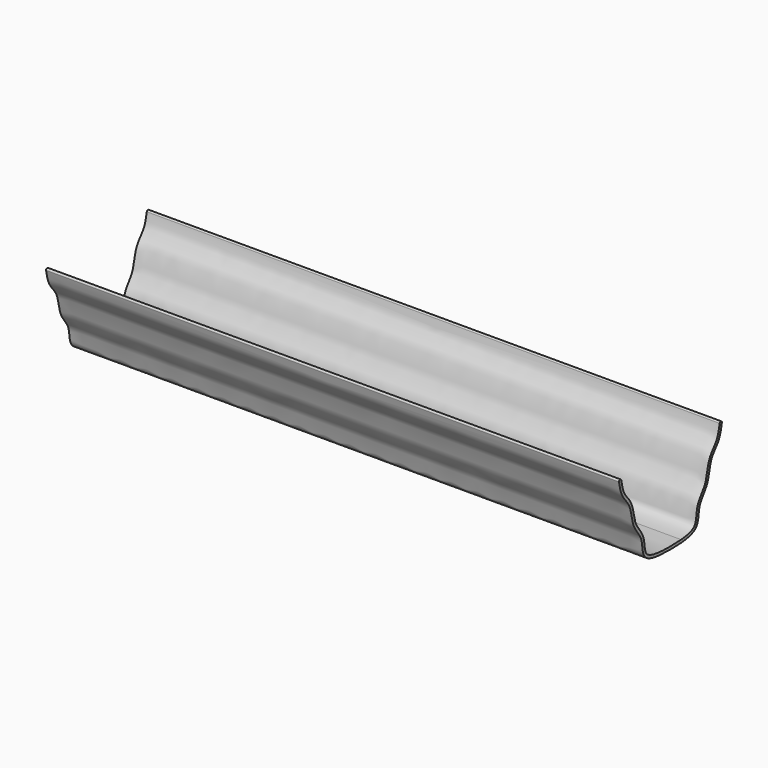
from build123d import *

# Parameters (mm, degrees)
F1_DEPTH = 610


# Not quite as in the source:
# - ends of sketch curves that miss each other by under 0.0002 mm in the source are joined
# - the dataset's text gives a spline's control points without its knots; the knots are read off the source's solid


with BuildPart() as f1:
    # F0 (on Right) → F1 (new body)
    with BuildSketch(Plane.YZ):
        with BuildLine():
            add(Edge.make_bspline(
                [(-6.5371447453, 100.0838043479), (-6.7706498844, 98.7103560222), (-7.2769413201, 95.966442744), (-8.2462300011, 91.9595019059), (-9.3037510376, 88.7948658007), (-10.3440569893, 86.4178038959), (-11.2307456768, 84.7238978183), (-12.2403989924, 83.1327544504), (-13.7314030487, 81.0971306843), (-15.7697396376, 78.6342860816), (-17.8019003352, 76.0598448924), (-19.2697771779, 73.7976975728), (-20.2543484515, 71.9667309835), (-21.0728069506, 69.9675927938), (-21.9644751836, 67.1317082104), (-22.8208505479, 63.3393291587), (-23.5880679523, 59.4204357255), (-24.2982442677, 56.3341514977), (-24.9152930999, 54.0757040586), (-25.5299125954, 52.2670731086), (-26.0987925353, 50.8798986568), (-26.7265419191, 49.5377250168), (-27.6192869804, 47.9259926379), (-28.8144352862, 46.0694225719), (-30.0870954542, 44.2604615596), (-31.3889305982, 42.4695513152), (-32.6711410298, 40.6663234118), (-33.8840399285, 38.8197513275), (-34.9770680963, 36.8983087952), (-35.7441787823, 35.2087841297), (-36.245684668, 33.7892000703), (-36.6603912488, 32.3205401383), (-37.0314295875, 30.4232254421), (-37.3426701, 28.0880308878), (-37.7016109413, 24.956073947), (-38.2751198805, 21.1168701085), (-39.5879465674, 17.6919434206), (-41.4132093167, 15.3464026837), (-43.884361824, 13.3003757024), (-48.4648476434, 11.3486413482), (-54.6911472323, 10.0868951516), (-58.9601875507, 9.6146321059), (-60.5720902436, 9.4757778746)],
                knots=[0, 0, 0, 0, 0.03125, 0.0625, 0.09375, 0.109375, 0.125, 0.140625, 0.15625, 0.1875, 0.21875, 0.234375, 0.25, 0.265625, 0.28125, 0.3125, 0.34375, 0.359375, 0.375, 0.390625, 0.3984375, 0.40625, 0.421875, 0.4375, 0.453125, 0.46875, 0.484375, 0.5, 0.515625, 0.53125, 0.5390625, 0.546875, 0.5625, 0.578125, 0.59375, 0.625, 0.65625, 0.671875, 0.6875, 0.71875, 0.75, 0.7681993638, 0.7681993638, 0.7681993638, 0.7681993638], degree=3))
            ThreePointArc((-6.5371447453, 100.0838043479), (-7.7645113289, 101.8139967008), (-9.4947036818, 100.5866301172))
            add(Edge.make_bspline(
                [(-9.4947036818, 100.5866301172), (-9.723489658, 99.2409393238), (-10.2154650316, 96.5775155495), (-10.984099453, 93.4060678093), (-11.7253161057, 91.0179222177), (-12.351032201, 89.3152360524), (-12.9364195699, 87.9786891729), (-13.445069822, 86.9641431497), (-13.8449752198, 86.237110404), (-14.2714951974, 85.5325548459), (-14.883703547, 84.6020829341), (-15.7352720489, 83.4380223818), (-16.8740485904, 82.0050765428), (-18.0941724522, 80.5130147466), (-19.3606115163, 78.9279555444), (-20.4182743502, 77.4990743402), (-21.2400483814, 76.2738452745), (-21.8370919113, 75.3102683333), (-22.4086512808, 74.2972930377), (-22.9492281356, 73.2237773821), (-23.4401123128, 72.1063379574), (-24.0242674729, 70.5860968403), (-24.6327831857, 68.64688946), (-25.2296829702, 66.2937826991), (-25.7451190854, 63.9292340336), (-26.2217625213, 61.5819904015), (-26.6985692792, 59.280556009), (-27.2107834687, 57.056451861), (-27.6926120569, 55.295580755), (-28.1236953584, 53.960179636), (-28.473009584, 52.9974452444), (-28.8479928364, 52.0836294372), (-29.3934828733, 50.9171718759), (-30.1894656071, 49.4774115594), (-31.2965609822, 47.7557860025), (-32.5198063414, 46.0161067231), (-33.8170759051, 44.2313930138), (-35.140653965, 42.37078801), (-36.43738975, 40.3984692762), (-37.4456660647, 38.6286705807), (-38.1730927218, 37.1189779146), (-38.5863632984, 36.1338877597), (-38.8873866246, 35.3191685524), (-39.0976860325, 34.6916248477), (-39.2882860981, 34.0554206664), (-39.5152977744, 33.2063939821), (-39.7518092025, 32.1482507218), (-40.0512888446, 30.478702112), (-40.3223470736, 28.4366280651), (-40.5908821572, 26.094352671), (-40.89399031, 23.9016800338), (-41.3011875448, 21.9112530753), (-41.8613191997, 20.1758141026), (-42.6066042503, 18.7044565974), (-43.4154210799, 17.6672121122), (-44.2460282782, 16.9035328467), (-44.9853969828, 16.3577743125), (-45.8907269157, 15.8235872099), (-46.9721354151, 15.3045309126), (-48.2104811138, 14.8152141046), (-50.0529843689, 14.2110000128), (-52.6812922381, 13.5577191822), (-56.2490599407, 12.9455882658), (-59.0331081681, 12.6252377637), (-60.5727693793, 12.4869516331), (-60.7761499105, 12.4693210267)],
                knots=[0, 0, 0, 0, 0.03125, 0.0625, 0.078125, 0.09375, 0.109375, 0.1171875, 0.125, 0.1328125, 0.140625, 0.15625, 0.171875, 0.1875, 0.203125, 0.21875, 0.2265625, 0.234375, 0.2421875, 0.25, 0.2578125, 0.265625, 0.28125, 0.296875, 0.3125, 0.328125, 0.34375, 0.359375, 0.375, 0.3828125, 0.390625, 0.3984375, 0.40625, 0.421875, 0.4375, 0.453125, 0.46875, 0.484375, 0.5, 0.515625, 0.5234375, 0.53125, 0.53515625, 0.5390625, 0.54296875, 0.546875, 0.5546875, 0.5625, 0.578125, 0.59375, 0.609375, 0.625, 0.640625, 0.65625, 0.671875, 0.6796875, 0.6875, 0.6953125, 0.703125, 0.7109375, 0.71875, 0.734375, 0.75, 0.765625, 0.7679922272, 0.7679922272, 0.7679922272, 0.7679922272], degree=3))
            add(Edge.make_bspline(
                [(-140.5052963182, 100.5866301172), (-140.276510342, 99.2409393238), (-139.7845349684, 96.5775155495), (-139.015900547, 93.4060678093), (-138.2746838943, 91.0179222177), (-137.648967799, 89.3152360524), (-137.0635804301, 87.9786891729), (-136.554930178, 86.9641431497), (-136.1550247802, 86.237110404), (-135.7285048026, 85.5325548459), (-135.116296453, 84.6020829341), (-134.2647279511, 83.4380223818), (-133.1259514096, 82.0050765428), (-131.9058275478, 80.5130147466), (-130.6393884837, 78.9279555444), (-129.5817256498, 77.4990743402), (-128.7599516186, 76.2738452745), (-128.1629080887, 75.3102683333), (-127.5913487192, 74.2972930377), (-127.0507718644, 73.2237773821), (-126.5598876872, 72.1063379574), (-125.9757325271, 70.5860968403), (-125.3672168143, 68.64688946), (-124.7703170298, 66.2937826991), (-124.2548809146, 63.9292340336), (-123.7782374787, 61.5819904015), (-123.3014307208, 59.280556009), (-122.7892165313, 57.056451861), (-122.3073879431, 55.295580755), (-121.8763046416, 53.960179636), (-121.526990416, 52.9974452444), (-121.1520071636, 52.0836294372), (-120.6065171267, 50.9171718759), (-119.8105343929, 49.4774115594), (-118.7034390178, 47.7557860025), (-117.4801936586, 46.0161067231), (-116.1829240949, 44.2313930138), (-114.859346035, 42.37078801), (-113.56261025, 40.3984692762), (-112.5543339353, 38.6286705807), (-111.8269072782, 37.1189779146), (-111.4136367016, 36.1338877597), (-111.1126133754, 35.3191685524), (-110.9023139675, 34.6916248477), (-110.7117139019, 34.0554206664), (-110.4847022256, 33.2063939821), (-110.2481907975, 32.1482507218), (-109.9487111554, 30.478702112), (-109.6776529264, 28.4366280651), (-109.4091178428, 26.094352671), (-109.10600969, 23.9016800338), (-108.6988124552, 21.9112530753), (-108.1386808003, 20.1758141026), (-107.3933957497, 18.7044565974), (-106.5845789201, 17.6672121122), (-105.7539717218, 16.9035328467), (-105.0146030172, 16.3577743125), (-104.1092730843, 15.8235872099), (-103.0278645849, 15.3045309126), (-101.7895188862, 14.8152141046), (-99.9470156311, 14.2110000128), (-97.3187077619, 13.5577191822), (-93.7509400593, 12.9455882658), (-89.8689345695, 12.4988997366), (-84.3935825665, 12.1034311284), (-77.2067630007, 11.9388633447), (-70.1126435589, 12.0750053269), (-64.809324713, 12.2759728551), (-62.201228655, 12.398488893), (-60.9005172536, 12.4631129163), (-60.7761499105, 12.4693210267)],
                knots=[0, 0, 0, 0, 0.03125, 0.0625, 0.078125, 0.09375, 0.109375, 0.1171875, 0.125, 0.1328125, 0.140625, 0.15625, 0.171875, 0.1875, 0.203125, 0.21875, 0.2265625, 0.234375, 0.2421875, 0.25, 0.2578125, 0.265625, 0.28125, 0.296875, 0.3125, 0.328125, 0.34375, 0.359375, 0.375, 0.3828125, 0.390625, 0.3984375, 0.40625, 0.421875, 0.4375, 0.453125, 0.46875, 0.484375, 0.5, 0.515625, 0.5234375, 0.53125, 0.53515625, 0.5390625, 0.54296875, 0.546875, 0.5546875, 0.5625, 0.578125, 0.59375, 0.609375, 0.625, 0.640625, 0.65625, 0.671875, 0.6796875, 0.6875, 0.6953125, 0.703125, 0.7109375, 0.71875, 0.734375, 0.75, 0.765625, 0.78125, 0.8125, 0.84375, 0.859375, 0.875, 0.8766615277, 0.8766615277, 0.8766615277, 0.8766615277], degree=3))
            ThreePointArc((-140.5052963182, 100.5866301172), (-142.2354886711, 101.8139967008), (-143.4628552547, 100.0838043479))
            add(Edge.make_bspline(
                [(-143.4628552547, 100.0838043479), (-143.2293501156, 98.7103560222), (-142.7230586799, 95.966442744), (-141.7537699989, 91.9595019059), (-140.6962489624, 88.7948658007), (-139.6559430107, 86.4178038959), (-138.7692543232, 84.7238978183), (-137.7596010076, 83.1327544504), (-136.2685969513, 81.0971306843), (-134.2302603624, 78.6342860816), (-132.1980996648, 76.0598448924), (-130.7302228221, 73.7976975728), (-129.7456515485, 71.9667309835), (-128.9271930494, 69.9675927938), (-128.0355248164, 67.1317082104), (-127.1791494521, 63.3393291587), (-126.4119320477, 59.4204357255), (-125.7017557323, 56.3341514977), (-125.0847069001, 54.0757040586), (-124.4700874046, 52.2670731086), (-123.9012074647, 50.8798986568), (-123.2734580809, 49.5377250168), (-122.3807130196, 47.9259926379), (-121.1855647138, 46.0694225719), (-119.9129045458, 44.2604615596), (-118.6110694018, 42.4695513152), (-117.3288589702, 40.6663234118), (-116.1159600715, 38.8197513275), (-115.0229319037, 36.8983087952), (-114.2558212177, 35.2087841297), (-113.754315332, 33.7892000703), (-113.3396087512, 32.3205401383), (-112.9685704125, 30.4232254421), (-112.6573299, 28.0880308878), (-112.2983890587, 24.956073947), (-111.7248801195, 21.1168701085), (-110.4120534326, 17.6919434206), (-108.5867906833, 15.3464026837), (-106.115638176, 13.3003757024), (-101.5351523566, 11.3486413482), (-94.301940604, 9.8828465711), (-85.9812891212, 9.1380434831), (-77.2034138309, 8.9381010647), (-70.0276489837, 9.0760424081), (-64.6807378705, 9.2786910878), (-62.0382645593, 9.4028348724), (-60.7148909827, 9.4686377045), (-60.5720902436, 9.4757778746)],
                knots=[0, 0, 0, 0, 0.03125, 0.0625, 0.09375, 0.109375, 0.125, 0.140625, 0.15625, 0.1875, 0.21875, 0.234375, 0.25, 0.265625, 0.28125, 0.3125, 0.34375, 0.359375, 0.375, 0.390625, 0.3984375, 0.40625, 0.421875, 0.4375, 0.453125, 0.46875, 0.484375, 0.5, 0.515625, 0.53125, 0.5390625, 0.546875, 0.5625, 0.578125, 0.59375, 0.625, 0.65625, 0.671875, 0.6875, 0.71875, 0.75, 0.78125, 0.8125, 0.84375, 0.859375, 0.875, 0.8769032209, 0.8769032209, 0.8769032209, 0.8769032209], degree=3))
        make_face()
    extrude(amount=F1_DEPTH)


solid = f1.part
